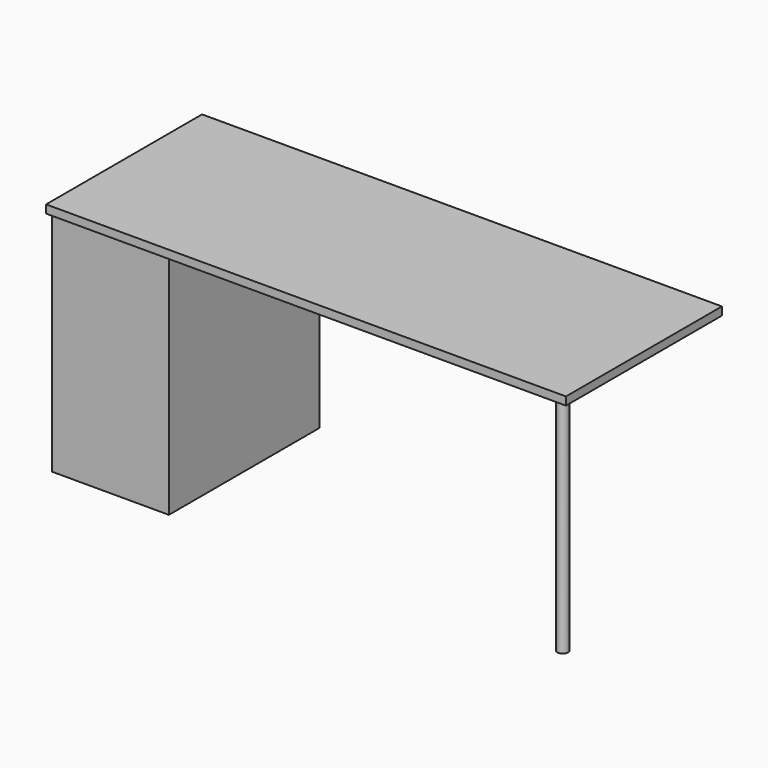
from build123d import *

# Parameters (mm, degrees)
F1_START = 700
F0_W     = 1600
F0_H     = 600
F1_DEPTH = 25
F2_W     = 360
F2_H     = 580
F3_DEPTH = 700
F4_R     = 16.35
F5_DEPTH = 700


# Not quite as in the source:
# - a feature names something its author has since deleted; it is built from what else it names


with BuildPart() as f1:
    # F0 (on Top) → F1 (new body)
    with BuildSketch(Plane.XY.offset(F1_START)):
        Rectangle(F0_W, F0_H)
    extrude(amount=F1_DEPTH)


with BuildPart() as f3:
    # F2 (on Top) → F3 (new body)
    with BuildSketch(Plane.XY):
        with Locations((-610, 0)):
            Rectangle(F2_W, F2_H)
    extrude(amount=F3_DEPTH)


with BuildPart() as f5:
    # F4 (on Top) → F5 (new body)
    with BuildSketch(Plane.XY):
        with Locations((750, -250)):
            Circle(F4_R)
    extrude(amount=F5_DEPTH)


solid = Compound([f1.part, f3.part, f5.part])
